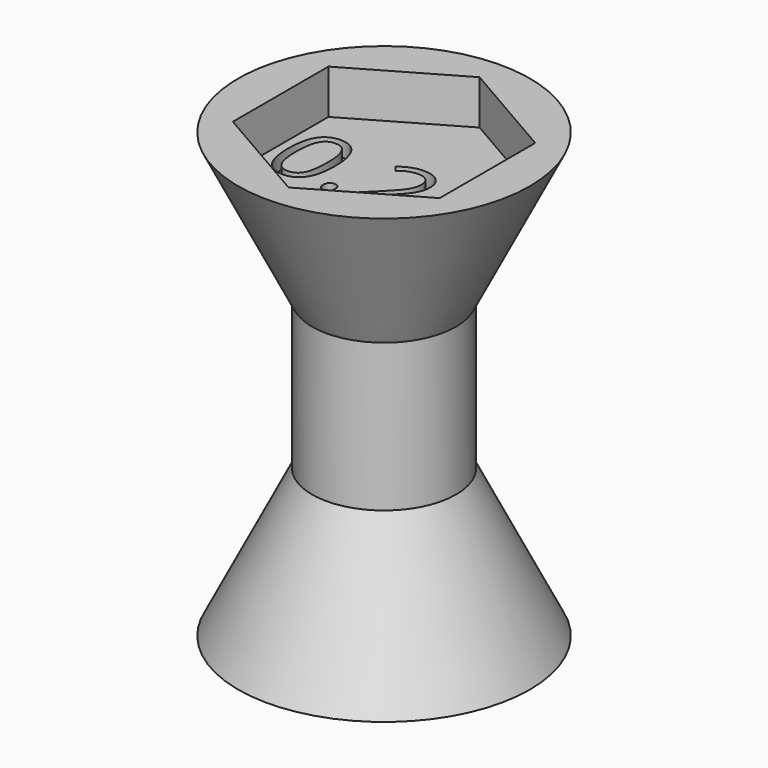
from build123d import *

# Parameters (mm, degrees)
F3_DEPTH     = 3
F4_TEXT_SIZE = 6.7887169011
F5_DEPTH     = 1


# Not quite as in the source:
# - Text() gives the source's letters only with a copy of the font that has no kerning and outlines rounded to 1/6400 em; it was checked with that copy


with BuildPart() as f1:
    # F0 (on Front) → F1 (revolve)
    with BuildSketch(Plane.XZ):
        Polygon((9.875, 15), (0, 15), (0, -15), (9.875, -15), (4.875, -5), (4.875, 5), align=None)
    revolve(axis=Axis((0, 0, 0), (0, 0, -1)))

    # F2 (on face) → F3 (cut)
    with BuildSketch(Plane.XY.offset(15)):
        Polygon((7, 4.0414518843), (0, 8.0829037687), (-7, 4.0414518843), (-7, -4.0414518843), (0, -8.0829037687), (7, -4.0414518843), align=None)
    extrude(amount=-F3_DEPTH, mode=Mode.SUBTRACT)

    # F4 (on face) → F5 (cut)
    with BuildSketch(Plane.XY.offset(12)):
        with Locations((-6.75, -2.5414518843)):
            Text('0.25', F4_TEXT_SIZE, font='Open Sans', text_align=(TextAlign.LEFT, TextAlign.BOTTOM))
    extrude(amount=-F5_DEPTH, mode=Mode.SUBTRACT)


solid = f1.part
